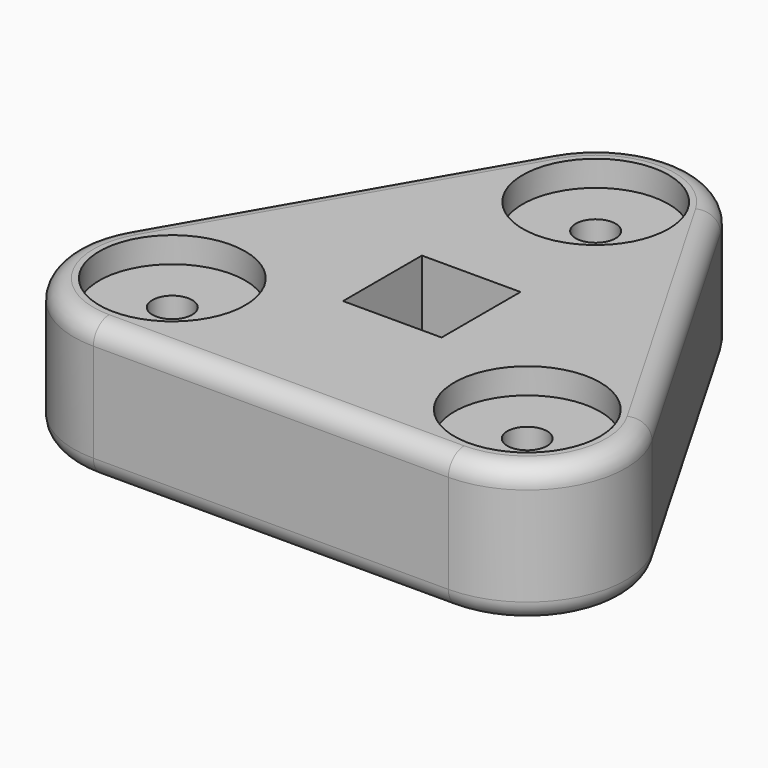
from build123d import *

# Parameters (mm, degrees)
F0_R          = 9.398
F2_DEPTH      = 17.78
F3_DEPTH      = 14.478
F1_W          = 12.7
F1_H          = 12.7
F4_DEPTH      = 107
F4_DEPTH_BACK = 17.781
F5_D          = 5.1308
F6_R          = 2.54
F7_R          = 2.54
F8_R          = 2.54
F9_R          = 5.08
F10_DEPTH     = 6.35


# Not quite as in the source:
# - an extrude ends at something that could not be found from the text; its depth is read off the source's solid


with BuildPart() as f2:
    # F0 (on Top) → F2 (new body)
    with BuildSketch(Plane.XY):
        with BuildLine():
            ThreePointArc((10.9985226281, 32.7464543073), (0, 39.0964543073), (-10.9985226281, 32.7464543073))
            Line((-10.9985226281, 32.7464543073), (-33.8585226281, -6.8482271537))
            ThreePointArc((-33.8585226281, -6.8482271537), (-33.8585226281, -19.5482271537), (-22.86, -25.8982271537))
            Line((-22.86, -25.8982271537), (22.86, -25.8982271537))
            ThreePointArc((22.86, -25.8982271537), (33.8585226281, -19.5482271537), (33.8585226281, -6.8482271537))
            Line((33.8585226281, -6.8482271537), (10.9985226281, 32.7464543073))
        make_face()
        with Locations((-22.86, -13.1982271537)):
            Circle(F0_R, mode=Mode.SUBTRACT)
        with Locations((22.86, -13.1982271537)):
            Circle(F0_R, mode=Mode.SUBTRACT)
        with Locations((0, 26.3964543073)):
            Circle(F0_R, mode=Mode.SUBTRACT)
    extrude(amount=F2_DEPTH)

    # F0 (on Top) → F3 (join)
    with BuildSketch(Plane.XY):
        with Locations((-22.86, -13.1982271537)):
            Circle(F0_R)
        with Locations((22.86, -13.1982271537)):
            Circle(F0_R)
        with Locations((0, 26.3964543073)):
            Circle(F0_R)
    extrude(amount=F3_DEPTH)

    # F1 (on face) → F4 (cut, two sides)
    with BuildSketch(Plane.XY) as f4_sk:
        Rectangle(F1_W, F1_H)
    extrude(amount=-F4_DEPTH, mode=Mode.SUBTRACT)
    extrude(f4_sk.sketch, amount=F4_DEPTH_BACK, mode=Mode.SUBTRACT)

    # F5 (through all)
    with Locations(Plane(origin=(0, 0, 0), x_dir=(1, 0, 0), z_dir=(0, 0, -1))):
        with Locations((-22.86, 13.1982271537), (22.86, 13.1982271537), (0, -26.3964543073)):
            Hole(F5_D / 2)

    # F6
    f6_edges = [f2.edges().sort_by_distance(p)[0] for p in [
        (-22.428523, 12.949114, 17.78),
    ]]
    fillet(f6_edges, radius=F6_R)

    # F7
    f7_edges = [f2.edges().sort_by_distance(p)[0] for p in [
        (22.428523, 12.949114, 0),
    ]]
    fillet(f7_edges, radius=F7_R)

    # F8
    f8_edges = [f2.edges().sort_by_distance(p)[0] for p in [
        (6.35, 0, 0),
        (0, -6.35, 0),
        (0, 6.35, 0),
        (-6.35, 0, 0),
    ]]
    fillet(f8_edges, radius=F8_R)

    # F9 (on face) → F10 (cut)
    with BuildSketch(Plane.XY):
        with Locations((22.86, -13.1982271537)):
            Circle(F9_R)
        with Locations((0, 26.3964543073)):
            Circle(F9_R)
        with Locations((-22.86, -13.1982271537)):
            Circle(F9_R)
    extrude(amount=F10_DEPTH, mode=Mode.SUBTRACT)


solid = f2.part
